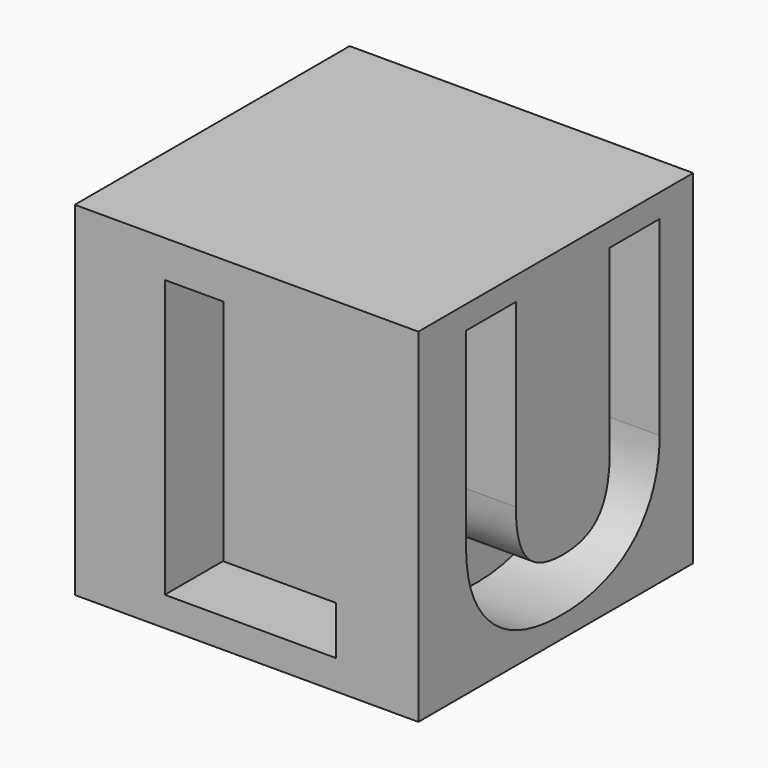
from build123d import *

# Parameters (mm, degrees)
F0_W         = 25.4
F0_H         = 25.4
F1_DEPTH     = 25.4
F2_TEXT_SIZE = 28.7029038494
F3_DEPTH     = 6.35
F4_TEXT_SIZE = 30.5324353071
F5_DEPTH     = 6.35
F6_TEXT_SIZE = 30.9238766527
F7_DEPTH     = 6.35
F8_TEXT_SIZE = 30.4541460031
F9_DEPTH     = 6.35


# Not quite as in the source:
# - Text() gives the source's letters only with a copy of the font that has no kerning and outlines rounded to 1/6400 em; it was checked with that copy


with BuildPart() as f1:
    # F0 (on Front) → F1 (new body)
    with BuildSketch(Plane.XZ):
        Rectangle(F0_W, F0_H)
    extrude(amount=F1_DEPTH)

    # F2 (on face) → F3 (cut)
    with BuildSketch(Plane.XZ.offset(25.4)):
        with Locations((-8.6266724393, -10.5226424057)):
            Text('L', F2_TEXT_SIZE, font='Open Sans', font_style=FontStyle.BOLD, text_align=(TextAlign.LEFT, TextAlign.BOTTOM))
    extrude(amount=-F3_DEPTH, mode=Mode.SUBTRACT)

    # F4 (on face) → F5 (cut)
    with BuildSketch(Plane.YZ.offset(12.7)):
        with Locations((-23.5910378397, -10.8239594847)):
            Text('U', F4_TEXT_SIZE, font='Open Sans', font_style=FontStyle.BOLD, text_align=(TextAlign.LEFT, TextAlign.BOTTOM))
    extrude(amount=-F5_DEPTH, mode=Mode.SUBTRACT)

    # F6 (on face) → F7 (cut)
    with BuildSketch(Plane(origin=(0, 0, 0), x_dir=(-1, 0, 0), z_dir=(0, 1, 0))):
        with Locations((-10.9480265528, -11.2793371081)):
            Text('K', F6_TEXT_SIZE, font='Open Sans', font_style=FontStyle.BOLD, text_align=(TextAlign.LEFT, TextAlign.BOTTOM))
    extrude(amount=-F7_DEPTH, mode=Mode.SUBTRACT)

    # F8 (on face) → F9 (cut)
    with BuildSketch(Plane(origin=(-12.7, 0, 0), x_dir=(0, -1, 0), z_dir=(-1, 0, 0))):
        with Locations((4.223817843, -10.866826633)):
            Text('E', F8_TEXT_SIZE, font='Open Sans', font_style=FontStyle.BOLD, text_align=(TextAlign.LEFT, TextAlign.BOTTOM))
    extrude(amount=-F9_DEPTH, mode=Mode.SUBTRACT)


solid = f1.part
